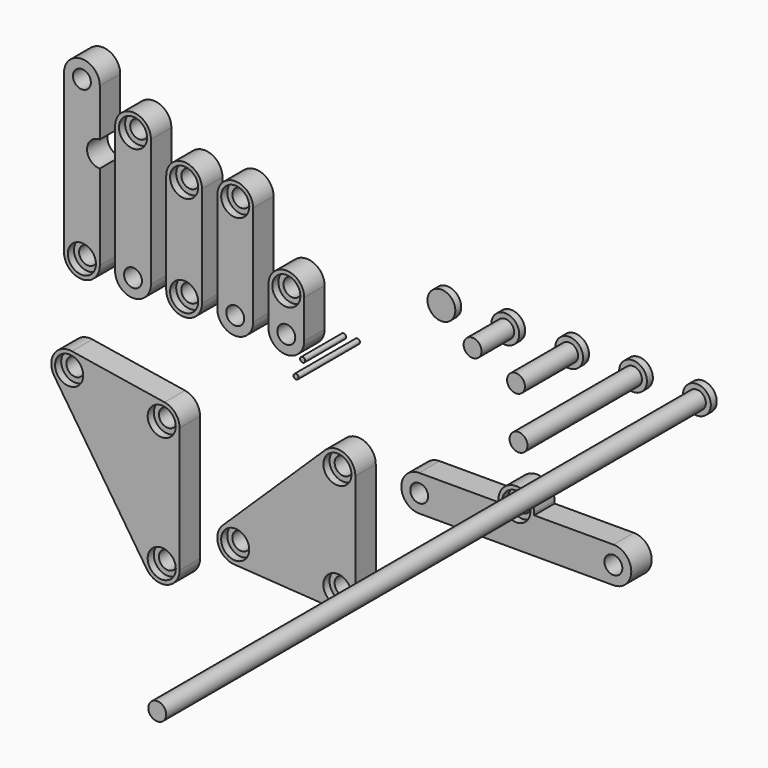
from build123d import *

# Parameters (mm, degrees)
F1_R      = 3.5
F2_DEPTH  = 10
F3_R      = 1
F4_DEPTH  = 20
F5_DEPTH  = 30
F7_DEPTH  = 10
F10_R     = 5.5
F10_R_2   = 3.5
F11_DEPTH = 3
F12_R     = 5.5
F12_R_2   = 3.5
F13_DEPTH = 3
F14_R     = 5.5
F14_R_2   = 3.5
F15_DEPTH = 3
F16_R     = 5.5
F17_DEPTH = 3
F18_R     = 5.5
F19_DEPTH = 3
F20_R     = 5.5
F20_R_2   = 3.5
F21_DEPTH = 3
F22_R     = 5.5
F23_DEPTH = 3
F24_R     = 5.45
F25_DEPTH = 2.9
F26_R     = 3.5
F27_DEPTH = 16
F28_DEPTH = 26
F29_DEPTH = 56
F30_DEPTH = 264
F31_R     = 5.5
F31_R_2   = 3.5
F32_DEPTH = 3
F33_R     = 5.5
F33_R_2   = 3.5
F34_DEPTH = 3
F35_R     = 3.5
F36_DEPTH = 2


# Not quite as in the source:
# - a feature names something its author has since deleted; it is built from what else it names


with BuildPart() as f2:
    # F1 (on Front) → F2 (new body)
    with BuildSketch(Plane.XZ):
        with BuildLine():
            Line((17, -81.5), (17, -40))
            ThreePointArc((17, -40), (12.7248098424, -33.5521002394), (5.1213110507, -34.9801997913))
            Line((5.1213110507, -34.9801997913), (-34.8936677561, -73.8703202732))
            ThreePointArc((-34.8936677561, -73.8703202732), (-36.5833416613, -81.3101637481), (-30.4705687475, -85.8752788771))
            Line((-30.4705687475, -85.8752788771), (9.5444100592, -88.4851583952))
            ThreePointArc((9.5444100592, -88.4851583952), (14.7859623073, -86.6082839382), (17, -81.5))
        make_face()
        with Locations((10, -81.5)):
            Circle(F1_R, mode=Mode.SUBTRACT)
        with Locations((-30.0149788067, -78.8901204819)):
            Circle(F1_R, mode=Mode.SUBTRACT)
        with Locations((10, -40)):
            Circle(F1_R, mode=Mode.SUBTRACT)
    extrude(amount=F2_DEPTH)

    # F16 (on face) → F17 (cut)
    with BuildSketch(Plane.XZ.offset(10)):
        with Locations((10, -40)):
            Circle(F16_R)
        with Locations((10, -81.5)):
            Circle(F16_R)
        with Locations((-30.0149788067, -78.8901204819)):
            Circle(F16_R)
    extrude(amount=-F17_DEPTH, mode=Mode.SUBTRACT)


with BuildPart() as f2b:
    # F1 (on Front) → F2, piece 2 (new body)
    with BuildSketch(Plane.XZ):
        with BuildLine():
            Line((-57.6548790335, -38.8900720763), (-93.8933437135, -33.0880312599))
            ThreePointArc((-93.8933437135, -33.0880312599), (-100.8832662527, -36.2069566045), (-100.838878017, -43.8610236341))
            Line((-100.838878017, -43.8610236341), (-64.6004133369, -98.6630644504))
            ThreePointArc((-64.6004133369, -98.6630644504), (-56.7456169336, -101.5054782226), (-51.76153532, -94.8020408163))
            Line((-51.76153532, -94.8020408163), (-51.76153532, -45.8020408163))
            ThreePointArc((-51.76153532, -45.8020408163), (-53.4348762354, -41.2603777952), (-57.6548790335, -38.8900720763))
        make_face()
        with Locations((-58.76153532, -94.8020408163)):
            Circle(F1_R, mode=Mode.SUBTRACT)
        with Locations((-95, -40)):
            Circle(F1_R, mode=Mode.SUBTRACT)
        with Locations((-58.76153532, -45.8020408163)):
            Circle(F1_R, mode=Mode.SUBTRACT)
    extrude(amount=F2_DEPTH)

    # F18 (on face) → F19 (cut)
    with BuildSketch(Plane.XZ.offset(10)):
        with Locations((-58.76153532, -45.8020408163)):
            Circle(F18_R)
        with Locations((-95, -40)):
            Circle(F18_R)
        with Locations((-58.76153532, -94.8020408163)):
            Circle(F18_R)
    extrude(amount=-F19_DEPTH, mode=Mode.SUBTRACT)


with BuildPart() as f2c:
    # F1 (on Front) → F2, piece 3 (new body)
    with BuildSketch(Plane.XZ):
        with BuildLine():
            Line((-97, 61.9), (-97, 0))
            ThreePointArc((-97, 0), (-90, -7), (-83, 0))
            Line((-83, 0), (-83, 61.9))
            ThreePointArc((-83, 61.9), (-90, 68.9), (-97, 61.9))
        make_face()
        with Locations((-90, 0)):
            Circle(F1_R, mode=Mode.SUBTRACT)
        with Locations((-90, 61.9)):
            Circle(F1_R, mode=Mode.SUBTRACT)
    extrude(amount=F2_DEPTH)

    # F6 (on face) → F7 (cut, through all)
    with BuildSketch(Plane.XZ.offset(10)):
        with BuildLine():
            Line((-83, 33.4), (-83, 43.4))
            ThreePointArc((-83, 43.4), (-88, 38.4), (-83, 33.4))
        make_face()
    extrude(amount=-F7_DEPTH, mode=Mode.SUBTRACT)

    # F20 (on face) → F21 (cut)
    with BuildSketch(Plane.XZ.offset(10)):
        with Locations((-90, 0)):
            Circle(F20_R)
        with Locations((-90, 0)):
            Circle(F20_R_2, mode=Mode.SUBTRACT)
    extrude(amount=-F21_DEPTH, mode=Mode.SUBTRACT)


with BuildPart() as f2d:
    # F1 (on Front) → F2, piece 4 (new body)
    with BuildSketch(Plane.XZ):
        with BuildLine():
            Line((-77, 50), (-77, 0))
            ThreePointArc((-77, 0), (-70, -7), (-63, 0))
            Line((-63, 0), (-63, 50))
            ThreePointArc((-63, 50), (-70, 57), (-77, 50))
        make_face()
        with Locations((-70, 0)):
            Circle(F1_R, mode=Mode.SUBTRACT)
        with Locations((-70, 50)):
            Circle(F1_R, mode=Mode.SUBTRACT)
    extrude(amount=F2_DEPTH)

    # F14 (on face) → F15 (cut)
    with BuildSketch(Plane.XZ.offset(10)):
        with Locations((-70, 50)):
            Circle(F14_R)
        with Locations((-70, 50)):
            Circle(F14_R_2, mode=Mode.SUBTRACT)
    extrude(amount=-F15_DEPTH, mode=Mode.SUBTRACT)


with BuildPart() as f2e:
    # F1 (on Front) → F2, piece 5 (new body)
    with BuildSketch(Plane.XZ):
        with BuildLine():
            Line((-57, 39.4), (-57, 0))
            ThreePointArc((-57, 0), (-50, -7), (-43, 0))
            Line((-43, 0), (-43, 39.4))
            ThreePointArc((-43, 39.4), (-50, 46.4), (-57, 39.4))
        make_face()
        with Locations((-50, 0)):
            Circle(F1_R, mode=Mode.SUBTRACT)
        with Locations((-50, 39.4)):
            Circle(F1_R, mode=Mode.SUBTRACT)
    extrude(amount=F2_DEPTH)

    # F22 (on face) → F23 (cut)
    with BuildSketch(Plane.XZ.offset(10)):
        with Locations((-50, 39.4)):
            Circle(F22_R)
        with Locations((-50, 0)):
            Circle(F22_R)
    extrude(amount=-F23_DEPTH, mode=Mode.SUBTRACT)


with BuildPart() as f2f:
    # F1 (on Front) → F2, piece 6 (new body)
    with BuildSketch(Plane.XZ):
        with BuildLine():
            Line((-37, 39.3), (-37, 0))
            ThreePointArc((-37, 0), (-30, -7), (-23, 0))
            Line((-23, 0), (-23, 39.3))
            ThreePointArc((-23, 39.3), (-30, 46.3), (-37, 39.3))
        make_face()
        with Locations((-30, 0)):
            Circle(F1_R, mode=Mode.SUBTRACT)
        with Locations((-30, 39.3)):
            Circle(F1_R, mode=Mode.SUBTRACT)
    extrude(amount=F2_DEPTH)

    # F31 (on face) → F32 (cut)
    with BuildSketch(Plane.XZ.offset(10)):
        with Locations((-30, 39.3)):
            Circle(F31_R)
        with Locations((-30, 39.3)):
            Circle(F31_R_2, mode=Mode.SUBTRACT)
    extrude(amount=-F32_DEPTH, mode=Mode.SUBTRACT)


with BuildPart() as f2g:
    # F1 (on Front) → F2, piece 7 (new body)
    with BuildSketch(Plane.XZ):
        with BuildLine():
            Line((73, -30.8), (42, -30.8))
            ThreePointArc((42, -30.8), (35, -37.8), (42, -44.8))
            Line((42, -44.8), (118, -44.8))
            ThreePointArc((118, -44.8), (125, -37.8), (118, -30.8))
            Line((118, -30.8), (87, -30.8))
            Line((87, -30.8), (87, -30))
            ThreePointArc((87, -30), (80, -23), (73, -30))
            Line((73, -30), (73, -30.8))
        make_face()
        with Locations((42, -37.8)):
            Circle(F1_R, mode=Mode.SUBTRACT)
        with Locations((118, -37.8)):
            Circle(F1_R, mode=Mode.SUBTRACT)
        with Locations((80, -30)):
            Circle(F1_R, mode=Mode.SUBTRACT)
    extrude(amount=F2_DEPTH)

    # F33 (on face) → F34 (cut)
    with BuildSketch(Plane.XZ.offset(10)):
        with Locations((80, -30)):
            Circle(F33_R)
        with Locations((80, -30)):
            Circle(F33_R_2, mode=Mode.SUBTRACT)
    extrude(amount=-F34_DEPTH, mode=Mode.SUBTRACT)


with BuildPart() as f2h:
    # F1 (on Front) → F2, piece 8 (new body)
    with BuildSketch(Plane.XZ):
        with BuildLine():
            Line((-3, 0), (-3, 15))
            ThreePointArc((-3, 15), (-10, 22), (-17, 15))
            Line((-17, 15), (-17, 0))
            ThreePointArc((-17, 0), (-10, -7), (-3, 0))
        make_face()
        with Locations((-10, 0)):
            Circle(F1_R, mode=Mode.SUBTRACT)
        with Locations((-10, 15)):
            Circle(F1_R, mode=Mode.SUBTRACT)
    extrude(amount=F2_DEPTH)

    # F10 (on face) → F11 (cut)
    with BuildSketch(Plane.XZ.offset(10)):
        with Locations((-10, 15)):
            Circle(F10_R)
        with Locations((-10, 15)):
            Circle(F10_R_2, mode=Mode.SUBTRACT)
    extrude(amount=-F11_DEPTH, mode=Mode.SUBTRACT)

    # F12 (on face) → F13 (cut)
    with BuildSketch(Plane(origin=(0, 0, 0), x_dir=(-1, 0, 0), z_dir=(0, 1, 0))):
        with Locations((10, 0)):
            Circle(F12_R)
        with Locations((10, 0)):
            Circle(F12_R_2, mode=Mode.SUBTRACT)
    extrude(amount=-F13_DEPTH, mode=Mode.SUBTRACT)


with BuildPart() as f4:
    # F3 (on Front) → F4 (new body)
    with BuildSketch(Plane.XZ):
        with Locations((4.3974108437, 0)):
            Circle(F3_R)
    extrude(amount=F4_DEPTH)


with BuildPart() as f5:
    # F3 (on Front) → F5 (new body)
    with BuildSketch(Plane.XZ):
        with Locations((9.7946263296, 0)):
            Circle(F3_R)
    extrude(amount=F5_DEPTH)


with BuildPart() as f25:
    # F24 (on Front) → F25 (new body)
    with BuildSketch(Plane.XZ):
        with Locations((45, 25)):
            Circle(F24_R)
    extrude(amount=F25_DEPTH)

    # F35 (on face) → F36 (cut)
    with BuildSketch(Plane(origin=(0, 0, 0), x_dir=(-1, 0, 0), z_dir=(0, 1, 0))):
        with Locations((-45, 25)):
            Circle(F35_R)
    extrude(amount=-F36_DEPTH, mode=Mode.SUBTRACT)


with BuildPart() as f25b:
    # F24 (on Front) → F25, piece 2 (new body)
    with BuildSketch(Plane.XZ):
        with Locations((70, 25)):
            Circle(F24_R)
    extrude(amount=F25_DEPTH)

    # F26 (on face) → F27 (join)
    with BuildSketch(Plane.XZ.offset(2.9)):
        with Locations((70, 25)):
            Circle(F26_R)
    extrude(amount=F27_DEPTH)


with BuildPart() as f25c:
    # F24 (on Front) → F25, piece 3 (new body)
    with BuildSketch(Plane.XZ):
        with Locations((95, 25)):
            Circle(F24_R)
    extrude(amount=F25_DEPTH)

    # F26 (on face) → F28 (join)
    with BuildSketch(Plane.XZ.offset(2.9)):
        with Locations((95, 25)):
            Circle(F26_R)
    extrude(amount=F28_DEPTH)


with BuildPart() as f25d:
    # F24 (on Front) → F25, piece 4 (new body)
    with BuildSketch(Plane.XZ):
        with Locations((120, 25)):
            Circle(F24_R)
    extrude(amount=F25_DEPTH)

    # F26 (on face) → F29 (join)
    with BuildSketch(Plane.XZ.offset(2.9)):
        with Locations((120, 25)):
            Circle(F26_R)
    extrude(amount=F29_DEPTH)


with BuildPart() as f25e:
    # F24 (on Front) → F25, piece 5 (new body)
    with BuildSketch(Plane.XZ):
        with Locations((145, 25)):
            Circle(F24_R)
    extrude(amount=F25_DEPTH)

    # F26 (on face) → F30 (join)
    with BuildSketch(Plane.XZ.offset(2.9)):
        with Locations((145, 25)):
            Circle(F26_R)
    extrude(amount=F30_DEPTH)


solid = Compound([f2.part, f2b.part, f2c.part, f2d.part, f2e.part, f2f.part, f2g.part, f2h.part, f4.part, f5.part, f25.part, f25b.part, f25c.part, f25d.part, f25e.part])
